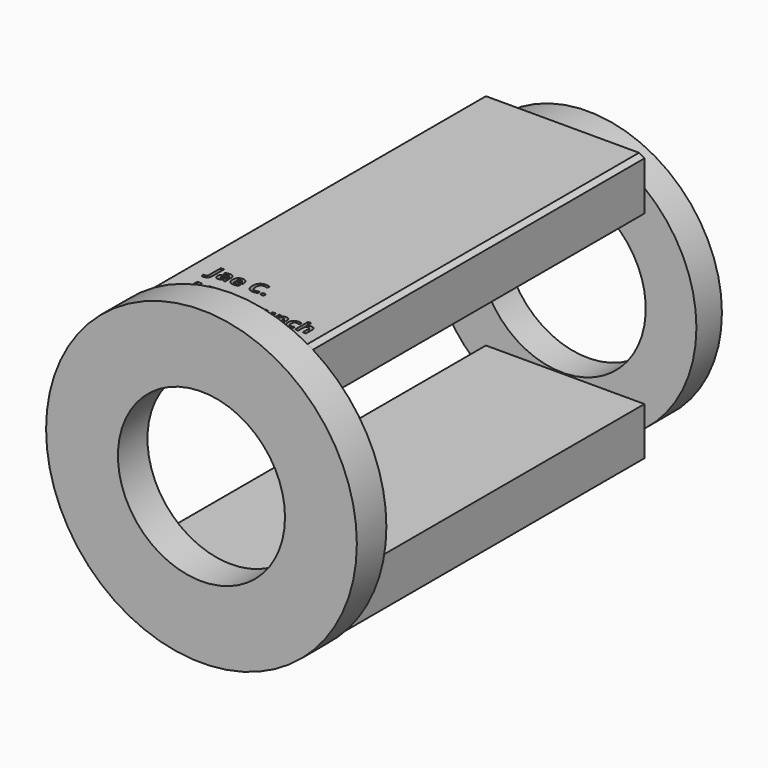
from build123d import *

# Parameters (mm, degrees)
F0_R         = 23.5279535521
F0_R_2       = 12.6488022349
F1_DEPTH     = 5.588
F2_W         = 24.0045808212
F2_H         = 7.2303343914
F3_DEPTH     = 62.738
F4_R         = 20.2853657258
F4_R_2       = 12.6129162171
F5_DEPTH     = 4.826
F6_TEXT_SIZE = 3.2667059643
F7_DEPTH     = 2.032


# Not quite as in the source:
# - Text() gives the source's letters only with a copy of the font that has no kerning and outlines rounded to 1/6400 em; it was checked with that copy


with BuildPart() as f1:
    # F0 (on Front) → F1 (new body)
    with BuildSketch(Plane.XZ):
        Circle(F0_R)
        Circle(F0_R_2, mode=Mode.SUBTRACT)
    extrude(amount=F1_DEPTH)

    # F2 (on face) → F3 (join)
    with BuildSketch(Plane(origin=(0, 0, 0), x_dir=(-1, 0, 0), z_dir=(0, 1, 0))):
        with BuildLine():
            Line((11.593216467, 12.6422736794), (11.593216467, 20.4734445148))
            Line((11.593216467, 20.4734445148), (-11.593216467, 20.4734445148))
            ThreePointArc((-11.593216467, 20.4734445148), (-12.0047438157, 20.2348887882), (-12.4113643542, 19.9880622677))
            Line((-12.4113643542, 19.9880622677), (-12.4113643542, 12.6422736794))
            Line((-12.4113643542, 12.6422736794), (-0.4063424596, 12.6422736794))
            ThreePointArc((-0.4063424596, 12.6422736794), (0, 12.6488022349), (0.4063424596, 12.6422736794))
            Line((0.4063424596, 12.6422736794), (11.593216467, 12.6422736794))
        make_face()
        with Locations((-0.4090739436, -16.372895072)):
            Rectangle(F2_W, F2_H)
    extrude(amount=F3_DEPTH)

    # F4 (on face) → F5 (join)
    with BuildSketch(Plane(origin=(0, 62.738, 0), x_dir=(-1, 0, 0), z_dir=(0, 1, 0))):
        Circle(F4_R)
        Circle(F4_R_2, mode=Mode.SUBTRACT)
    extrude(amount=F5_DEPTH)

    # F6 (on face) → F7 (cut)
    with BuildSketch(Plane.XY.offset(20.4734445148)):
        with Locations((-8.8476760294, 6.4381930749)):
            Text('Jae C.', F6_TEXT_SIZE, font='Open Sans', font_style=FontStyle.BOLD, text_align=(TextAlign.LEFT, TextAlign.BOTTOM))
        with Locations((-8.8476760294, 1.9954729634)):
            Text('MIT Launch', F6_TEXT_SIZE, font='Open Sans', font_style=FontStyle.BOLD, text_align=(TextAlign.LEFT, TextAlign.BOTTOM))
    extrude(amount=-F7_DEPTH, mode=Mode.SUBTRACT)


solid = f1.part
